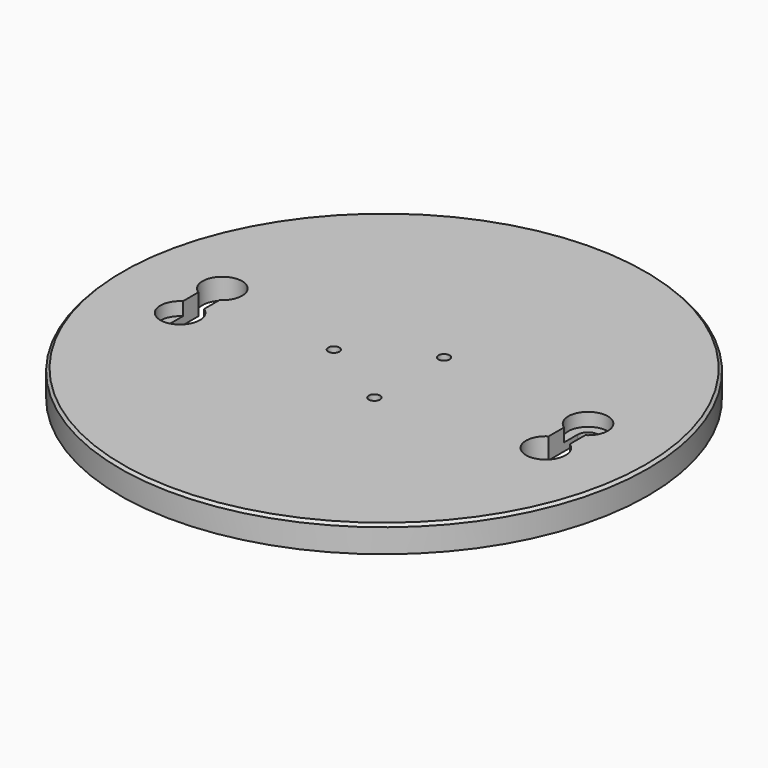
from build123d import *

# Parameters (mm, degrees)
F0_R     = 63.5
F0_R_2   = 57.15
F0_R_3   = 1.3462
F1_DEPTH = 6.35
F2_START = 3.175
F2_DEPTH = 3.175
F3_SIZE  = 0.635
F4_DEPTH = 1.27


with BuildPart() as f1:
    # F0 (on Top) → F1 (new body)
    with BuildSketch(Plane.XY):
        Circle(F0_R)
        Circle(F0_R_2, mode=Mode.SUBTRACT)
        Circle(F0_R_2)
        with Locations((6.0491874454, -10.4775)):
            Circle(F0_R_3, mode=Mode.SUBTRACT)
        with BuildLine():
            ThreePointArc((-41.4540905122, -2.3213766309), (-39.8240691544, -4.0494939415), (-39.2315905122, -6.35))
            ThreePointArc((-39.2315905122, -6.35), (-46.2945965707, -10.5200213579), (-46.5340905122, -2.3213766309))
            Line((-46.5340905122, -2.3213766309), (-46.5340905122, 2.3213766309))
            ThreePointArc((-46.5340905122, 2.3213766309), (-46.2945965707, 10.5200213579), (-39.2315905122, 6.35))
            ThreePointArc((-39.2315905122, 6.35), (-39.8240691544, 4.0494939415), (-41.4540905122, 2.3213766309))
            Line((-41.4540905122, 2.3213766309), (-41.4540905122, -2.3213766309))
        make_face(mode=Mode.SUBTRACT)
        with Locations((-12.0983748909, 0)):
            Circle(F0_R_3, mode=Mode.SUBTRACT)
        with Locations((6.0491874454, 10.4775)):
            Circle(F0_R_3, mode=Mode.SUBTRACT)
        with BuildLine():
            ThreePointArc((48.7565905122, 6.35), (48.1641118701, 4.0494939415), (46.5340905122, 2.3213766309))
            Line((46.5340905122, 2.3213766309), (46.5340905122, -2.3213766309))
            ThreePointArc((46.5340905122, -2.3213766309), (48.1641118701, -4.0494939415), (48.7565905122, -6.35))
            ThreePointArc((48.7565905122, -6.35), (41.6935844538, -10.5200213579), (41.4540905122, -2.3213766309))
            Line((41.4540905122, -2.3213766309), (41.4540905122, 2.3213766309))
            ThreePointArc((41.4540905122, 2.3213766309), (41.6935844538, 10.5200213579), (48.7565905122, 6.35))
        make_face(mode=Mode.SUBTRACT)
        with BuildLine():
            ThreePointArc((-46.5340905122, -2.3213766309), (-46.2945965707, -10.5200213579), (-39.2315905122, -6.35))
            ThreePointArc((-39.2315905122, -6.35), (-39.8240691544, -4.0494939415), (-41.4540905122, -2.3213766309))
            Line((-41.4540905122, -2.3213766309), (-41.4540905122, -6.35))
            ThreePointArc((-41.4540905122, -6.35), (-43.9940905122, -8.89), (-46.5340905122, -6.35))
            Line((-46.5340905122, -6.35), (-46.5340905122, -2.3213766309))
        make_face()
        with BuildLine():
            ThreePointArc((41.4540905122, 6.35), (43.9940905122, 8.89), (46.5340905122, 6.35))
            Line((46.5340905122, 6.35), (46.5340905122, 2.3213766309))
            ThreePointArc((46.5340905122, 2.3213766309), (48.1641118701, 4.0494939415), (48.7565905122, 6.35))
            ThreePointArc((48.7565905122, 6.35), (41.6935844538, 10.5200213579), (41.4540905122, 2.3213766309))
            Line((41.4540905122, 2.3213766309), (41.4540905122, 6.35))
        make_face()
    extrude(amount=F1_DEPTH)

    # F0 (on Top) → F2 (cut)
    with BuildSketch(Plane.XY.offset(F2_START)):
        with BuildLine():
            ThreePointArc((-46.5340905122, -2.3213766309), (-46.2945965707, -10.5200213579), (-39.2315905122, -6.35))
            ThreePointArc((-39.2315905122, -6.35), (-39.8240691544, -4.0494939415), (-41.4540905122, -2.3213766309))
            Line((-41.4540905122, -2.3213766309), (-41.4540905122, -6.35))
            ThreePointArc((-41.4540905122, -6.35), (-43.9940905122, -8.89), (-46.5340905122, -6.35))
            Line((-46.5340905122, -6.35), (-46.5340905122, -2.3213766309))
        make_face()
        with BuildLine():
            Line((-41.4540905122, -6.35), (-41.4540905122, -2.3213766309))
            ThreePointArc((-41.4540905122, -2.3213766309), (-43.9940905122, -1.5875), (-46.5340905122, -2.3213766309))
            Line((-46.5340905122, -2.3213766309), (-46.5340905122, -6.35))
            ThreePointArc((-46.5340905122, -6.35), (-43.9940905122, -3.81), (-41.4540905122, -6.35))
        make_face()
        with BuildLine():
            Line((46.5340905122, 2.3213766309), (46.5340905122, 6.35))
            ThreePointArc((46.5340905122, 6.35), (43.9940905122, 3.81), (41.4540905122, 6.35))
            Line((41.4540905122, 6.35), (41.4540905122, 2.3213766309))
            ThreePointArc((41.4540905122, 2.3213766309), (43.9940905122, 1.5875), (46.5340905122, 2.3213766309))
        make_face()
        with BuildLine():
            ThreePointArc((41.4540905122, 6.35), (43.9940905122, 8.89), (46.5340905122, 6.35))
            Line((46.5340905122, 6.35), (46.5340905122, 2.3213766309))
            ThreePointArc((46.5340905122, 2.3213766309), (48.1641118701, 4.0494939415), (48.7565905122, 6.35))
            ThreePointArc((48.7565905122, 6.35), (41.6935844538, 10.5200213579), (41.4540905122, 2.3213766309))
            Line((41.4540905122, 2.3213766309), (41.4540905122, 6.35))
        make_face()
    extrude(amount=F2_DEPTH, mode=Mode.SUBTRACT)

    # F3
    f3_edges = [f1.edges().sort_by_distance(p)[0] for p in [
        (-63.5, 0, 6.35),
    ]]
    chamfer(f3_edges, length=F3_SIZE)

    # F0 (on Top) → F4 (cut)
    with BuildSketch(Plane.XY):
        Circle(F0_R_2)
        with Locations((6.0491874454, -10.4775)):
            Circle(F0_R_3, mode=Mode.SUBTRACT)
        with BuildLine():
            ThreePointArc((-41.4540905122, -2.3213766309), (-39.8240691544, -4.0494939415), (-39.2315905122, -6.35))
            ThreePointArc((-39.2315905122, -6.35), (-46.2945965707, -10.5200213579), (-46.5340905122, -2.3213766309))
            Line((-46.5340905122, -2.3213766309), (-46.5340905122, 2.3213766309))
            ThreePointArc((-46.5340905122, 2.3213766309), (-46.2945965707, 10.5200213579), (-39.2315905122, 6.35))
            ThreePointArc((-39.2315905122, 6.35), (-39.8240691544, 4.0494939415), (-41.4540905122, 2.3213766309))
            Line((-41.4540905122, 2.3213766309), (-41.4540905122, -2.3213766309))
        make_face(mode=Mode.SUBTRACT)
        with Locations((-12.0983748909, 0)):
            Circle(F0_R_3, mode=Mode.SUBTRACT)
        with Locations((6.0491874454, 10.4775)):
            Circle(F0_R_3, mode=Mode.SUBTRACT)
        with BuildLine():
            ThreePointArc((48.7565905122, 6.35), (48.1641118701, 4.0494939415), (46.5340905122, 2.3213766309))
            Line((46.5340905122, 2.3213766309), (46.5340905122, -2.3213766309))
            ThreePointArc((46.5340905122, -2.3213766309), (48.1641118701, -4.0494939415), (48.7565905122, -6.35))
            ThreePointArc((48.7565905122, -6.35), (41.6935844538, -10.5200213579), (41.4540905122, -2.3213766309))
            Line((41.4540905122, -2.3213766309), (41.4540905122, 2.3213766309))
            ThreePointArc((41.4540905122, 2.3213766309), (41.6935844538, 10.5200213579), (48.7565905122, 6.35))
        make_face(mode=Mode.SUBTRACT)
        with BuildLine():
            ThreePointArc((-46.5340905122, -2.3213766309), (-46.2945965707, -10.5200213579), (-39.2315905122, -6.35))
            ThreePointArc((-39.2315905122, -6.35), (-39.8240691544, -4.0494939415), (-41.4540905122, -2.3213766309))
            Line((-41.4540905122, -2.3213766309), (-41.4540905122, -6.35))
            ThreePointArc((-41.4540905122, -6.35), (-43.9940905122, -8.89), (-46.5340905122, -6.35))
            Line((-46.5340905122, -6.35), (-46.5340905122, -2.3213766309))
        make_face()
        with BuildLine():
            ThreePointArc((41.4540905122, 6.35), (43.9940905122, 8.89), (46.5340905122, 6.35))
            Line((46.5340905122, 6.35), (46.5340905122, 2.3213766309))
            ThreePointArc((46.5340905122, 2.3213766309), (48.1641118701, 4.0494939415), (48.7565905122, 6.35))
            ThreePointArc((48.7565905122, 6.35), (41.6935844538, 10.5200213579), (41.4540905122, 2.3213766309))
            Line((41.4540905122, 2.3213766309), (41.4540905122, 6.35))
        make_face()
    extrude(amount=F4_DEPTH, mode=Mode.SUBTRACT)


solid = f1.part
